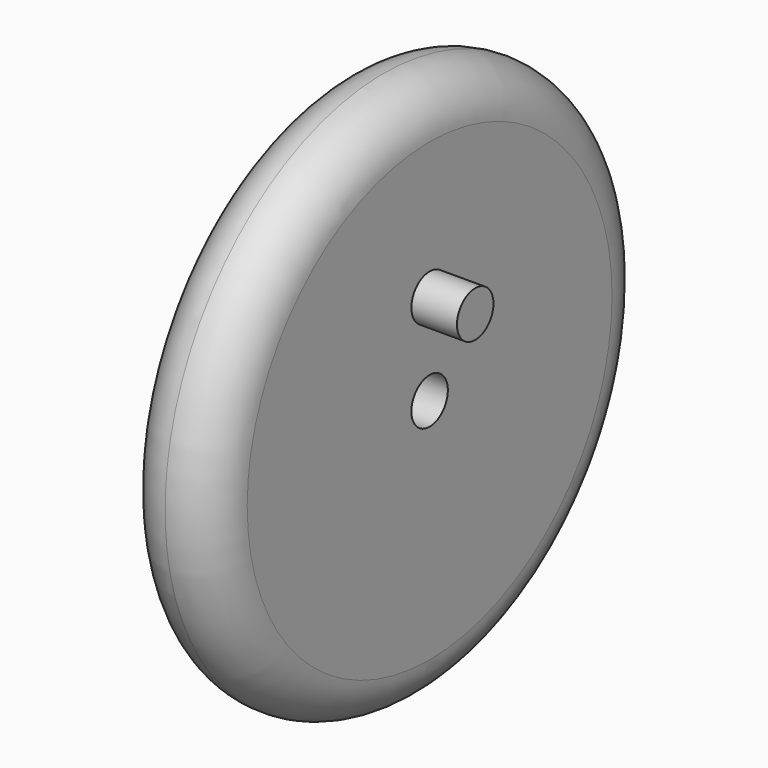
from build123d import *

# Parameters (mm, degrees)
F0_R     = 19.05
F3_DEPTH = 6.35
F2_R     = 1.5875
F4_DEPTH = 6.35
F5_R     = 3.175
F6_R     = 3.17499
F7_R     = 1.5875
F8_DEPTH = 3.175


# Not quite as in the source:
# - a fillet or chamfer is up to 0.001 mm smaller than in the source, because OpenCascade refuses the exact size


with BuildPart() as f3:
    # F0 (on Right) → F3 (new body)
    with BuildSketch(Plane.YZ):
        Circle(F0_R)
    extrude(amount=F3_DEPTH)

    # F2 (on face) → F4 (cut)
    with BuildSketch(Plane.YZ):
        Circle(F2_R)
    extrude(amount=F4_DEPTH, mode=Mode.SUBTRACT)

    # F5
    f5_edges = [f3.edges().sort_by_distance(p)[0] for p in [
        (0, -19.05, 0),
    ]]
    fillet(f5_edges, radius=F5_R)

    # F6 (radius 3.175 in the source; OpenCascade refuses exactly that, so slightly less here)
    f6_edges = [f3.edges().sort_by_distance(p)[0] for p in [
        (6.35, -19.05, 0),
    ]]
    fillet(f6_edges, radius=F6_R)

    # F7 (on face) → F8 (join)
    with BuildSketch(Plane.YZ.offset(6.35)):
        with Locations((0, 6.35)):
            Circle(F7_R)
    extrude(amount=F8_DEPTH)


solid = f3.part
